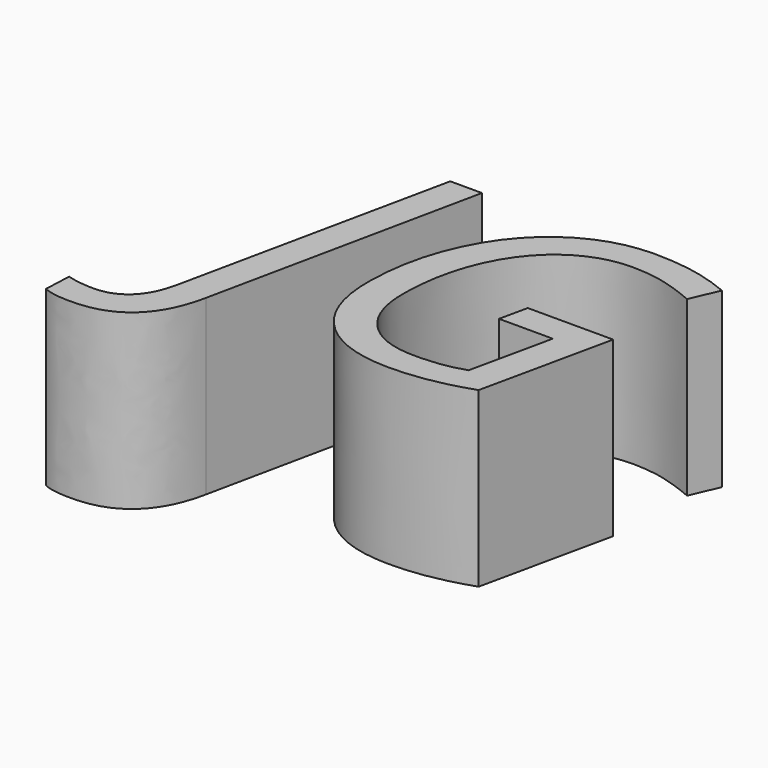
from build123d import *

# Parameters (mm, degrees)
F0_TEXT_SIZE = 16.7806218896
F1_DEPTH     = 7.62


# Not quite as in the source:
# - Text() gives the source's letters only with a copy of the font that has no kerning and outlines rounded to 1/6400 em; it was checked with that copy


with BuildPart() as f1:
    # F0 (on Top) → F1 (new body)
    with BuildSketch(Plane.XY):
        with Locations((-17.0491114259, 10.336862877)):
            Text('JG', F0_TEXT_SIZE, font='Open Sans', font_style=FontStyle.ITALIC, text_align=(TextAlign.LEFT, TextAlign.BOTTOM))
    extrude(amount=F1_DEPTH)


solid = f1.part
